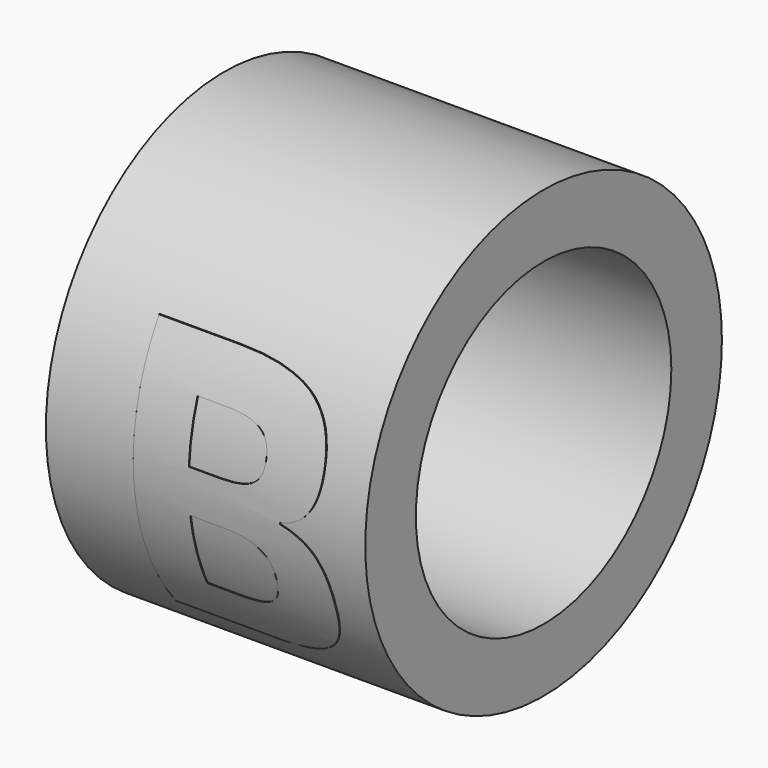
from build123d import *

# Parameters (mm, degrees)
F0_R         = 1.75
F0_R_2       = 1.745
F0_R_3       = 1.25
F1_DEPTH     = 2.5
F2_TEXT_SIZE = 2.8570699214
F3_REACH     = 4.2902588838
F4_DEPTH     = 2.5


# Not quite as in the source:
# - Text() gives the source's letters only with a copy of the font that has no kerning and outlines rounded to 1/6400 em; it was checked with that copy


with BuildPart() as f1:
    # F0 (on Right) → F1 (new body)
    with BuildSketch(Plane.YZ):
        Circle(F0_R)
        Circle(F0_R_2, mode=Mode.SUBTRACT)
        Circle(F0_R_2)
        Circle(F0_R_3, mode=Mode.SUBTRACT)
    extrude(amount=F1_DEPTH)

    f3_end = f1.faces().sort_by_distance((1.25, -1.75, 0))[0]
    # F2 (on Front) → F3 (intersect, up to a face of the model that its end follows)
    with BuildSketch(Plane.XZ):
        with Locations((0.4309935612, -1.1343103251)):
            Text('B', F2_TEXT_SIZE, font='Open Sans', font_style=FontStyle.BOLD, text_align=(TextAlign.LEFT, TextAlign.BOTTOM))
    f3_long = extrude(amount=F3_REACH, mode=Mode.PRIVATE)
    add(split(f3_long, bisect_by=f3_end, keep=Keep.BOTTOM, mode=Mode.PRIVATE), mode=Mode.INTERSECT)


with BuildPart() as f4:
    # F0 (on Right) → F4 (new body)
    with BuildSketch(Plane.YZ):
        Circle(F0_R_2)
        Circle(F0_R_3, mode=Mode.SUBTRACT)
    extrude(amount=F4_DEPTH)


solid = Compound([f1.part, f4.part])
